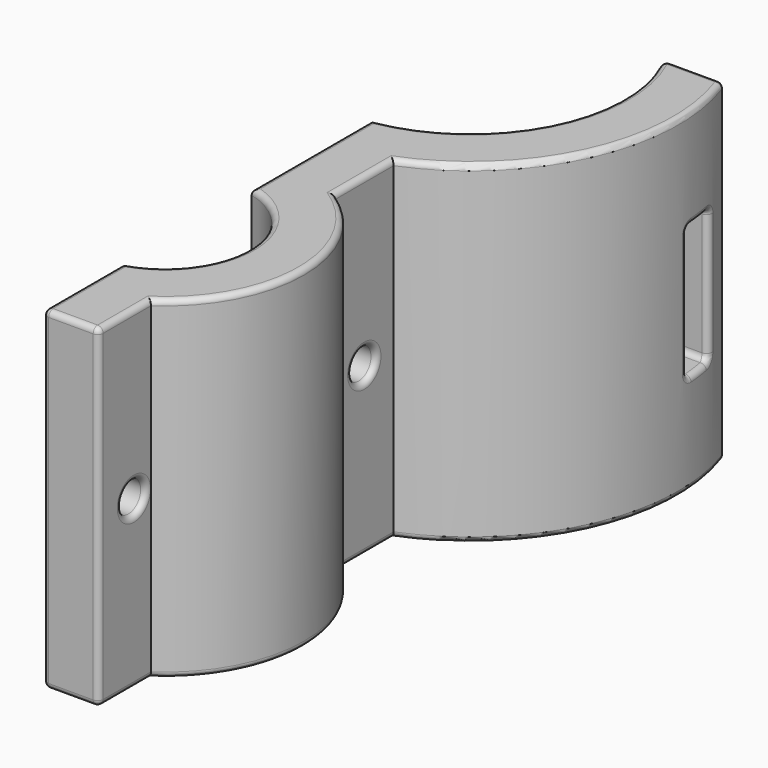
from build123d import *

# Parameters (mm, degrees)
F1_DEPTH = 38.1
F2_R     = 1.75
F3_DEPTH = 6.35
F4_W     = 3.81
F4_H     = 15.24
F5_DEPTH = 23.8135
F6_R     = 1.75
F7_DEPTH = 6.351000172
F8_R     = 0.635


with BuildPart() as f1:
    # F0 (on Top) → F1 (new body)
    with BuildSketch(Plane.XY):
        with BuildLine():
            ThreePointArc((15.4469541779, 51.7462283529), (15.5705240089, 35.6963257432), (2.54, 26.3250885072))
            Line((2.54, 26.3250885072), (2.54, 9.1800885072))
            ThreePointArc((2.54, 9.1800885072), (9.525, 0), (2.54, -9.1800885072))
            Line((2.54, -9.1800885072), (2.54, -20.6100885072))
            Line((2.54, -20.6100885072), (8.890000172, -20.6100885072))
            Line((8.890000172, -20.6100885072), (8.890000172, -13.1523200213))
            ThreePointArc((8.890000172, -13.1523200213), (15.875, 1.038e-07), (8.89, 13.1523201375))
            Line((8.89, 13.1523201375), (8.89, 21.5110824807))
            ThreePointArc((8.89, 21.5110824807), (21.7471476529, 33.9015270357), (22.3764305325, 51.7462283529))
            Line((22.3764305325, 51.7462283529), (15.4469541779, 51.7462283529))
        make_face()
    extrude(amount=-F1_DEPTH)

    # F2 (on face) → F3 (cut, through all)
    with BuildSketch(Plane.YZ.offset(8.89)):
        with Locations((17.3317013091, -19.05)):
            Circle(F2_R)
    extrude(amount=-F3_DEPTH, mode=Mode.SUBTRACT)

    # F4 (on Right) → F5 (cut, through all)
    with BuildSketch(Plane.YZ):
        with Locations((46.6662283529, -19.05)):
            Rectangle(F4_W, F4_H)
    extrude(amount=F5_DEPTH, mode=Mode.SUBTRACT)

    # F6 (on face) → F7 (cut, through all)
    with BuildSketch(Plane.YZ.offset(8.890000172)):
        with Locations((-15.5805000213, -19.05)):
            Circle(F6_R)
    extrude(amount=-F7_DEPTH, mode=Mode.SUBTRACT)

    # F8
    f8_edges = [f1.edges().sort_by_distance(p)[0] for p in [
        (18.911692, 51.746228, 0),
        (15.570524, 35.696326, 0),
        (2.54, 17.752589, 0),
        (9.525, 0, 0),
        (2.54, -14.895089, 0),
        (5.715, -20.610089, 0),
        (8.89, -16.881204, 0),
        (15.875, 0, 0),
        (8.89, 17.331701, 0),
        (21.747148, 33.901527, 0),
        (18.911692, 51.746228, -38.1),
        (15.570524, 35.696326, -38.1),
        (2.54, 17.752589, -38.1),
        (9.525, 0, -38.1),
        (2.54, -14.895089, -38.1),
        (5.715, -20.610089, -38.1),
        (8.89, -16.881204, -38.1),
        (15.875, 0, -38.1),
        (8.89, 17.331701, -38.1),
        (21.747148, 33.901527, -38.1),
        (2.54, -20.610089, -19.05),
        (8.89, -20.610089, -19.05),
        (22.376431, 51.746228, -19.05),
        (15.446954, 51.746228, -19.05),
        (5.715, 19.081701, -19.05),
        (8.89, 15.581701, -19.05),
        (2.54, 15.581701, -19.05),
        (8.89, -17.3305, -19.05),
        (5.715, -13.8305, -19.05),
        (2.54, -17.3305, -19.05),
        (17.188131, 46.685224, -11.43),
        (20.604116, 44.761228, -11.43),
        (23.613203, 46.676249, -11.43),
        (20.014356, 48.571228, -11.43),
        (17.188131, 46.685224, -26.67),
        (20.014356, 48.571228, -26.67),
        (23.613203, 46.676249, -26.67),
        (20.604116, 44.761228, -26.67),
        (23.288209, 48.571228, -19.05),
        (23.784261, 44.761228, -19.05),
        (17.423972, 44.761228, -19.05),
        (16.740502, 48.571228, -19.05),
    ]]
    fillet(f8_edges, radius=F8_R)


solid = f1.part
